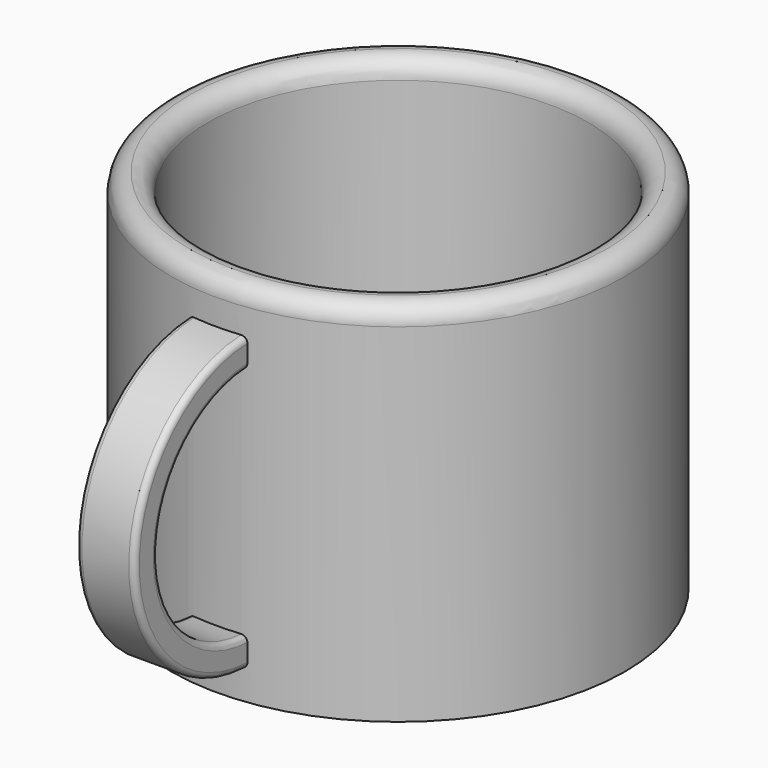
from build123d import *

# Parameters (mm, degrees)
F0_R     = 15.5
F1_DEPTH = 25
F2_T     = -2.5
F3_R     = 1.24999
F5_W     = 4
F5_H     = 2
F6_ANGLE = 180
F7_R     = 0.4


# Not quite as in the source:
# - a fillet or chamfer is up to 0.001 mm smaller than in the source, because OpenCascade refuses the exact size


with BuildPart() as f1:
    # F0 (on Top) → F1 (new body)
    with BuildSketch(Plane.XY):
        Circle(F0_R)
    extrude(amount=F1_DEPTH)

    # F2
    f2_openings = [f1.faces().sort_by_distance(p)[0] for p in [
        (0, 0, 25),
    ]]
    offset(amount=F2_T, openings=f2_openings)

    # F3 (radius 1.25 in the source; OpenCascade refuses exactly that, so slightly less here)
    f3_edges = [f1.edges().sort_by_distance(p)[0] for p in [
        (-15.5, 0, 25),
        (-13, 0, 25),
    ]]
    fillet(f3_edges, radius=F3_R)

    # F5 (on offset) → F6 (revolve)
    with BuildSketch(Plane.XZ.offset(15)):
        with Locations((0, 21)):
            Rectangle(F5_W, F5_H)
    revolve(axis=Axis((1, -15, 12), (1, 0, 0)), revolution_arc=F6_ANGLE)

    # F7
    f7_edges = [f1.edges().sort_by_distance(p)[0] for p in [
        (2, -25, 12),
        (-2, -25, 12),
        (2, -23, 12),
        (-2, -23, 12),
    ]]
    fillet(f7_edges, radius=F7_R)


solid = f1.part
